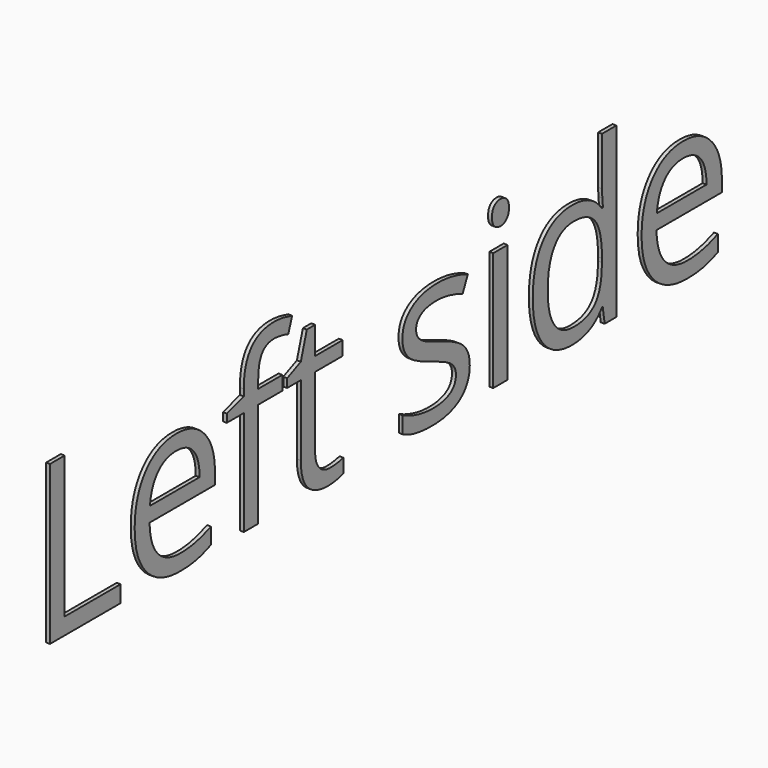
from build123d import *

# Parameters (mm, degrees)
F3_TEXT_SIZE = 1443.531198634
F4_DEPTH     = 25.4


# Not quite as in the source:
# - Text() gives the source's letters only with a copy of the font that has no kerning and outlines rounded to 1/6400 em; it was checked with that copy


with BuildPart() as f4:
    # F3 (on face) → F4 (new body)
    with BuildSketch(Plane.YZ):
        with Locations((-726.5051007271, -475.8520126343)):
            Text('Left side', F3_TEXT_SIZE, font='Open Sans', text_align=(TextAlign.LEFT, TextAlign.BOTTOM))
    extrude(amount=F4_DEPTH)


solid = f4.part
